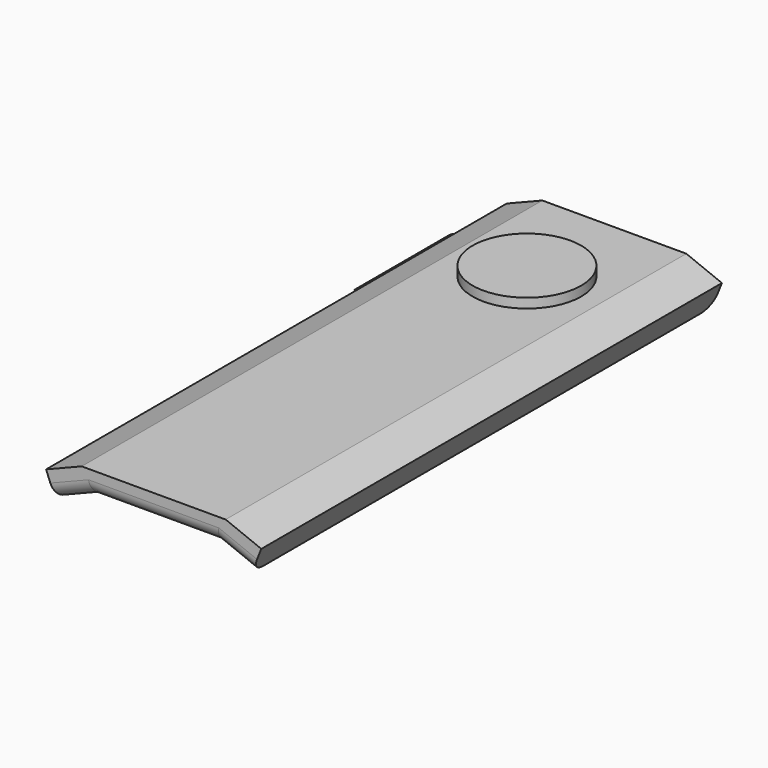
from build123d import *

# Parameters (mm, degrees)
F0_W       = 38.1
F0_H       = 152.4
F1_DEPTH   = 6.35
F2_SIZE2   = 2.53999
F2_SIZE    = 6.34999
F2_2_SIZE2 = 2.53999
F2_2_SIZE  = 6.34999
F3_W       = 152.4
F3_H       = 6.8391593051
F4_DEPTH   = 10.16
F5_W       = 152.4
F5_H       = 6.8391593051
F6_DEPTH   = 10.16
F7_R       = 3.81
F8_W       = 31.75
F8_H       = 5.08
F9_DEPTH   = 6.35
F10_W      = 4.318
F10_H      = 26.67
F11_DEPTH  = 25.4
F12_R      = 1.016
F13_R      = 14.3701538506
F14_DEPTH  = 2.54


# Not quite as in the source:
# - a fillet or chamfer is up to 0.001 mm smaller than in the source, because OpenCascade refuses the exact size


with BuildPart() as f1:
    # F0 (on Top) → F1 (new body)
    with BuildSketch(Plane.XY):
        with Locations((0.2864310518, 39.6771576124)):
            Rectangle(F0_W, F0_H)
    extrude(amount=F1_DEPTH)

    # F2 (size 6.35 and 2.54 in the source; OpenCascade refuses exactly that, so slightly less here)
    f2_edges = [f1.edges().sort_by_distance(p)[0] for p in [
        (-18.763569, 39.677158, 0),
    ]]
    f2_side = f1.faces().sort_by_distance((-18.763569, 39.677158, 3.175))[0]
    chamfer(f2_edges, length=F2_SIZE, length2=F2_SIZE2, reference=f2_side)

    # F2#2 (size 6.35 and 2.54 in the source; OpenCascade refuses exactly that, so slightly less here)
    f2_2_edges = [f1.edges().sort_by_distance(p)[0] for p in [
        (19.336431, 39.677158, 0),
    ]]
    f2_2_side = f1.faces().sort_by_distance((19.336431, 39.677158, 3.175))[0]
    chamfer(f2_2_edges, length=F2_2_SIZE, length2=F2_2_SIZE2, reference=f2_2_side)

    # F3 (on face) → F4 (join)
    with BuildSketch(Plane(origin=(-13.9858353002, 0, -5.5943341201), x_dir=(0, -1, 0), z_dir=(-0.9284766909, 0, -0.3713906764))):
        with Locations((-39.6771576124, 9.4448618971)):
            Rectangle(F3_W, F3_H)
    extrude(amount=F4_DEPTH)

    # F5 (on face) → F6 (join)
    with BuildSketch(Plane(origin=(14.4796819412, 0, -5.7918727765), x_dir=(0, 1, 0), z_dir=(0.9284766909, 0, -0.3713906764))):
        with Locations((39.6771576124, 9.6576175412)):
            Rectangle(F5_W, F5_H)
    extrude(amount=F6_DEPTH)

    # F7
    f7_edges = [f1.edges().sort_by_distance(p)[0] for p in [
        (0.286431, -36.522842, 0),
        (-20.940231, -36.522842, -1.886665),
        (21.513093, -36.522842, -1.886665),
        (21.513093, 115.877158, -1.886665),
        (0.286431, 115.877158, 0),
        (-20.940231, 115.877158, -1.886665),
    ]]
    fillet(f7_edges, radius=F7_R)

    # F8 (on face) → F9 (join)
    with BuildSketch(Plane(origin=(-23.4191584796, 0, -9.3676633918), x_dir=(0, -1, 0), z_dir=(-0.9284766909, 0, -0.3713906764))):
        with Locations((-87.9551129937, 8.5652822446)):
            Rectangle(F8_W, F8_H)
    extrude(amount=F9_DEPTH)

    # F10 (on face) → F11 (cut)
    with BuildSketch(Plane(origin=(-4.1243982839, 0, 10.3109957098), x_dir=(0.9284766909, 0, 0.3713906764), z_dir=(-0.3713906764, 0, 0.9284766909))):
        with Locations((-27.3822056114, 87.9551129937)):
            Rectangle(F10_W, F10_H)
    extrude(amount=-F11_DEPTH, mode=Mode.SUBTRACT)

    # F12
    f12_edges = [f1.edges().sort_by_distance(p)[0] for p in [
        (-31.552719, 87.955113, -0.660333),
        (-29.666054, 87.955113, -5.376994),
    ]]
    fillet(f12_edges, radius=F12_R)

    # F13 (on face) → F14 (join)
    with BuildSketch(Plane.XY.offset(6.35)):
        with Locations((0, 87.3177349567)):
            Circle(F13_R)
    extrude(amount=F14_DEPTH)


solid = f1.part
